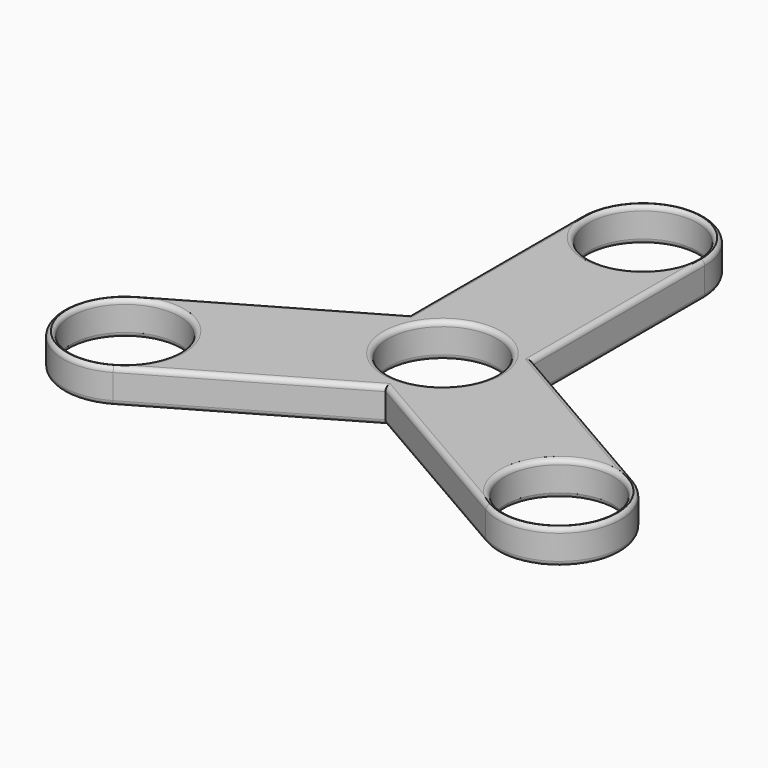
from build123d import *

# Parameters (mm, degrees)
F2_DEPTH      = 7
F1_R          = 11
F3_DEPTH      = 25.4
F4_T8_DEPTH   = 46.0831216351
F4_T13_DEPTH  = 46.0831216351
F4_T18_DEPTH  = 46.0831216351
F4_T23_DEPTH  = 46.0831216351
F4_T28_DEPTH  = 46.0831216351
F4_T37_DEPTH  = 46.0831216351
F4_T42_DEPTH  = 46.0831216351
F4_T51_DEPTH  = 46.0831216351
F4_T56_DEPTH  = 46.0831216351
F4_T59_ANGLE  = 180
F4_T61_ANGLE  = 180
F4_T63_ANGLE  = 180
F4_T67_DEPTH  = 46.0831216351
F4_T70_ANGLE  = 180
F4_T74_DEPTH  = 46.0831216351
F4_T77_ANGLE  = 180
F4_T81_DEPTH  = 46.0831216351
F4_T84_ANGLE  = 180
F4_T89_DEPTH  = 46.0831216351
F4_T93_DEPTH  = 46.0831216351
F4_T100_DEPTH = 46.0831216351
F4_T104_DEPTH = 46.0831216351
F4_T111_DEPTH = 46.0831216351
F4_T115_DEPTH = 46.0831216351
F4_T122_DEPTH = 46.0831216351
F4_T126_DEPTH = 46.0831216351
F4_T133_DEPTH = 46.0831216351
F4_T137_DEPTH = 46.0831216351
F4_T144_DEPTH = 46.0831216351
F4_T148_DEPTH = 46.0831216351
F5_R          = 1


# Not quite as in the source:
# - a fillet or chamfer that OpenCascade refuses, or shapes differently, is made with other operations: its cross-section is extruded or revolved along the edge and cut away or added


with BuildPart() as f2:
    # F0 (on Top) → F2 (new body)
    with BuildSketch(Plane.XY):
        with BuildLine():
            ThreePointArc((12.5, 50.8), (0, 63.3), (-12.5, 50.8))
            Line((-12.5, 50.8), (-12.5, 7.2168783649))
            Line((-12.5, 7.2168783649), (-50.2440905122, -14.5746824527))
            ThreePointArc((-50.2440905122, -14.5746824527), (-54.8194080596, -31.65), (-37.7440905122, -36.2253175473))
            Line((-37.7440905122, -36.2253175473), (0, -14.4337567297))
            Line((0, -14.4337567297), (37.7440905122, -36.2253175473))
            ThreePointArc((37.7440905122, -36.2253175473), (54.8194080596, -31.65), (50.2440905122, -14.5746824527))
            Line((50.2440905122, -14.5746824527), (12.5, 7.2168783649))
            Line((12.5, 7.2168783649), (12.5, 50.8))
        make_face()
    extrude(amount=F2_DEPTH)

    # F1 (on Top) → F3 (cut)
    with BuildSketch(Plane.XY):
        with Locations((0, 50.8)):
            Circle(F1_R)
        with Locations((-43.9940905122, -25.4)):
            Circle(F1_R)
        with Locations((43.9940905122, -25.4)):
            Circle(F1_R)
        Circle(F1_R)
    extrude(amount=F3_DEPTH, mode=Mode.SUBTRACT)

    # F4: fillet of radius 1 on 15 edges, made by hand

    # F4_s1 → F4_t2 (revolve, cut)
    with BuildSketch(Plane.XZ.offset(-50.8)):
        with BuildLine():
            ThreePointArc((12, 7), (11.2928932188, 6.7071067812), (11, 6))
            Line((11, 6), (11, 7))
            Line((11, 7), (12, 7))
        make_face()
    revolve(axis=Axis((0, 50.8, 7), (0, 0, -1)), mode=Mode.SUBTRACT)

    # F4_s3 → F4_t4 (revolve, cut)
    with BuildSketch(Plane.XZ.offset(-50.8)):
        with BuildLine():
            ThreePointArc((12, 0), (11.2928932188, 0.2928932188), (11, 1))
            Line((11, 1), (11, 0))
            Line((11, 0), (12, 0))
        make_face()
    revolve(axis=Axis((0, 50.8, 0), (0, 0, 1)), mode=Mode.SUBTRACT)


with BuildPart() as f4_tool6:
    # F4_s7 → F4_t8 (new body)
    with BuildSketch(Plane.XZ.offset(-50.8)):
        with BuildLine():
            ThreePointArc((-11.5, 0), (-12.2071067812, 0.2928932188), (-12.5, 1))
            Line((-12.5, 1), (-12.5, 0))
            Line((-12.5, 0), (-11.5, 0))
        make_face()
    extrude(amount=F4_T8_DEPTH)

    split(bisect_by=Plane(origin=(-6.25, 10.8253175473, 0), x_dir=(0, 0, 1), z_dir=(-0.5, 0.8660254038, 0)), keep=Keep.TOP)


with BuildPart() as f2_1:
    add(f2.part)

    # F4_t5: cut F4_tool6
    add(f4_tool6.part, mode=Mode.SUBTRACT)


with BuildPart() as f4_tool11:
    # F4_s12 → F4_t13 (new body)
    with BuildSketch(Plane.XZ.offset(-4.7168783649)):
        with BuildLine():
            ThreePointArc((11.5, 0), (12.2071067812, 0.2928932188), (12.5, 1))
            Line((12.5, 1), (12.5, 0))
            Line((12.5, 0), (11.5, 0))
        make_face()
    extrude(amount=-F4_T13_DEPTH)

    split(bisect_by=Plane(origin=(6.25, 10.8253175473, 0), x_dir=(0, 0, 1), z_dir=(0.5, 0.8660254038, 0)), keep=Keep.TOP)


with BuildPart() as f2_2:
    add(f2_1.part)

    # F4_t10: cut F4_tool11
    add(f4_tool11.part, mode=Mode.SUBTRACT)


with BuildPart() as f4_tool16:
    # F4_s17 → F4_t18 (new body)
    with BuildSketch(Plane.XZ.offset(-4.7168783649)):
        with BuildLine():
            ThreePointArc((11.5, 7), (12.2071067812, 6.7071067812), (12.5, 6))
            Line((12.5, 6), (12.5, 7))
            Line((12.5, 7), (11.5, 7))
        make_face()
    extrude(amount=-F4_T18_DEPTH)

    split(bisect_by=Plane(origin=(6.25, 10.8253175473, 0), x_dir=(0, 0, 1), z_dir=(0.5, 0.8660254038, 0)), keep=Keep.TOP)


with BuildPart() as f2_3:
    add(f2_2.part)

    # F4_t15: cut F4_tool16
    add(f4_tool16.part, mode=Mode.SUBTRACT)


with BuildPart() as f4_tool21:
    # F4_s22 → F4_t23 (new body)
    with BuildSketch(Plane(origin=(-4.0849364905, -2.3584391824, 0), x_dir=(0, 0, 1), z_dir=(-0.8660254038, -0.5, 0))):
        with BuildLine():
            ThreePointArc((0, 11.5), (0.2928932188, 12.2071067812), (1, 12.5))
            Line((1, 12.5), (0, 12.5))
            Line((0, 12.5), (0, 11.5))
        make_face()
    extrude(amount=F4_T23_DEPTH)

    split(bisect_by=Plane.YZ.offset(-12.5), keep=Keep.BOTTOM)


with BuildPart() as f2_4:
    add(f2_3.part)

    # F4_t20: cut F4_tool21
    add(f4_tool21.part, mode=Mode.SUBTRACT)


with BuildPart() as f4_tool26:
    # F4_s27 → F4_t28 (new body)
    with BuildSketch(Plane(origin=(-4.0849364905, -2.3584391824, 0), x_dir=(0, 0, 1), z_dir=(-0.8660254038, -0.5, 0))):
        with BuildLine():
            ThreePointArc((7, 11.5), (6.7071067812, 12.2071067812), (6, 12.5))
            Line((6, 12.5), (7, 12.5))
            Line((7, 12.5), (7, 11.5))
        make_face()
    extrude(amount=F4_T28_DEPTH)

    split(bisect_by=Plane.YZ.offset(-12.5), keep=Keep.BOTTOM)


with BuildPart() as f2_5:
    add(f2_4.part)

    # F4_t25: cut F4_tool26
    add(f4_tool26.part, mode=Mode.SUBTRACT)

    # F4_s30 → F4_t31 (revolve, cut)
    with BuildSketch(Plane.XZ.offset(25.4)):
        with BuildLine():
            ThreePointArc((-31.9940905122, 0), (-32.7011972934, 0.2928932188), (-32.9940905122, 1))
            Line((-32.9940905122, 1), (-32.9940905122, 0))
            Line((-32.9940905122, 0), (-31.9940905122, 0))
        make_face()
    revolve(axis=Axis((-43.9940905122, -25.4, 0), (0, 0, 1)), mode=Mode.SUBTRACT)

    # F4_s32 → F4_t33 (revolve, cut)
    with BuildSketch(Plane.XZ.offset(25.4)):
        with BuildLine():
            ThreePointArc((-31.9940905122, 7), (-32.7011972934, 6.7071067812), (-32.9940905122, 6))
            Line((-32.9940905122, 6), (-32.9940905122, 7))
            Line((-32.9940905122, 7), (-31.9940905122, 7))
        make_face()
    revolve(axis=Axis((-43.9940905122, -25.4, 7), (0, 0, -1)), mode=Mode.SUBTRACT)


with BuildPart() as f4_tool35:
    # F4_s36 → F4_t37 (new body)
    with BuildSketch(Plane(origin=(43.9940905122, -25.4, 0), x_dir=(0, 0, 1), z_dir=(-0.8660254038, 0.5, 0))):
        with BuildLine():
            ThreePointArc((7, 11.5), (6.7071067812, 12.2071067812), (6, 12.5))
            Line((6, 12.5), (7, 12.5))
            Line((7, 12.5), (7, 11.5))
        make_face()
    extrude(amount=F4_T37_DEPTH)

    split(bisect_by=Plane.YZ.offset(12.5), keep=Keep.TOP)


with BuildPart() as f2_6:
    add(f2_5.part)

    # F4_t34: cut F4_tool35
    add(f4_tool35.part, mode=Mode.SUBTRACT)


with BuildPart() as f4_tool40:
    # F4_s41 → F4_t42 (new body)
    with BuildSketch(Plane(origin=(4.0849364905, -2.3584391824, 0), x_dir=(0, 0, 1), z_dir=(0.8660254038, -0.5, 0))):
        with BuildLine():
            ThreePointArc((6, 12.5), (6.7071067812, 12.2071067812), (7, 11.5))
            Line((7, 11.5), (7, 12.5))
            Line((7, 12.5), (6, 12.5))
        make_face()
    extrude(amount=F4_T42_DEPTH)

    split(bisect_by=Plane(origin=(6.25, -10.8253175473, 0), x_dir=(0, 0, 1), z_dir=(0.5, -0.8660254038, 0)), keep=Keep.TOP)


with BuildPart() as f2_7:
    add(f2_6.part)

    # F4_t39: cut F4_tool40
    add(f4_tool40.part, mode=Mode.SUBTRACT)

    # F4_s44 → F4_t45 (revolve, cut)
    with BuildSketch(Plane.XZ.offset(25.4)):
        with BuildLine():
            ThreePointArc((55.9940905122, 7), (55.2869837311, 6.7071067812), (54.9940905122, 6))
            Line((54.9940905122, 6), (54.9940905122, 7))
            Line((54.9940905122, 7), (55.9940905122, 7))
        make_face()
    revolve(axis=Axis((43.9940905122, -25.4, 7), (0, 0, -1)), mode=Mode.SUBTRACT)

    # F4_s46 → F4_t47 (revolve, cut)
    with BuildSketch(Plane.XZ.offset(25.4)):
        with BuildLine():
            ThreePointArc((55.9940905122, 0), (55.2869837311, 0.2928932188), (54.9940905122, 1))
            Line((54.9940905122, 1), (54.9940905122, 0))
            Line((54.9940905122, 0), (55.9940905122, 0))
        make_face()
    revolve(axis=Axis((43.9940905122, -25.4, 0), (0, 0, 1)), mode=Mode.SUBTRACT)


with BuildPart() as f4_tool49:
    # F4_s50 → F4_t51 (new body)
    with BuildSketch(Plane(origin=(4.0849364905, -2.3584391824, 0), x_dir=(0, 0, 1), z_dir=(0.8660254038, -0.5, 0))):
        with BuildLine():
            ThreePointArc((1, 12.5), (0.2928932188, 12.2071067812), (0, 11.5))
            Line((0, 11.5), (0, 12.5))
            Line((0, 12.5), (1, 12.5))
        make_face()
    extrude(amount=F4_T51_DEPTH)

    split(bisect_by=Plane(origin=(6.25, -10.8253175473, 0), x_dir=(0, 0, 1), z_dir=(0.5, -0.8660254038, 0)), keep=Keep.TOP)


with BuildPart() as f2_8:
    add(f2_7.part)

    # F4_t48: cut F4_tool49
    add(f4_tool49.part, mode=Mode.SUBTRACT)


with BuildPart() as f4_tool54:
    # F4_s55 → F4_t56 (new body)
    with BuildSketch(Plane(origin=(43.9940905122, -25.4, 0), x_dir=(0, 0, 1), z_dir=(-0.8660254038, 0.5, 0))):
        with BuildLine():
            ThreePointArc((0, 11.5), (0.2928932188, 12.2071067812), (1, 12.5))
            Line((1, 12.5), (0, 12.5))
            Line((0, 12.5), (0, 11.5))
        make_face()
    extrude(amount=F4_T56_DEPTH)

    split(bisect_by=Plane.YZ.offset(12.5), keep=Keep.TOP)


with BuildPart() as f2_9:
    add(f2_8.part)

    # F4_t53: cut F4_tool54
    add(f4_tool54.part, mode=Mode.SUBTRACT)

    # F4_s58 → F4_t59 (revolve, cut)
    with BuildSketch(Plane(origin=(43.9940905122, -25.4, 0), x_dir=(0, 0, 1), z_dir=(-0.8660254038, 0.5, 0))):
        with BuildLine():
            ThreePointArc((0, -11.5), (0.2928932188, -12.2071067812), (1, -12.5))
            Line((1, -12.5), (0, -12.5))
            Line((0, -12.5), (0, -11.5))
        make_face()
    revolve(axis=Axis((43.9940905122, -25.4, 0), (0, 0, 1)), revolution_arc=F4_T59_ANGLE, mode=Mode.SUBTRACT)

    # F4_s60 → F4_t61 (revolve, cut)
    with BuildSketch(Plane(origin=(43.9940905122, -25.4, 0), x_dir=(0, 0, 1), z_dir=(-0.8660254038, 0.5, 0))):
        with BuildLine():
            ThreePointArc((7, -11.5), (6.7071067812, -12.2071067812), (6, -12.5))
            Line((6, -12.5), (7, -12.5))
            Line((7, -12.5), (7, -11.5))
        make_face()
    revolve(axis=Axis((43.9940905122, -25.4, 7), (0, 0, 1)), revolution_arc=F4_T61_ANGLE, mode=Mode.SUBTRACT)

    # F4_s62 → F4_t63 (revolve, cut)
    with BuildSketch(Plane(origin=(-43.9940905122, -25.4, 0), x_dir=(0, 0, 1), z_dir=(0.8660254038, 0.5, 0))):
        with BuildLine():
            ThreePointArc((6, -12.5), (6.7071067812, -12.2071067812), (7, -11.5))
            Line((7, -11.5), (7, -12.5))
            Line((7, -12.5), (6, -12.5))
        make_face()
    revolve(axis=Axis((-43.9940905122, -25.4, 7), (0, 0, 1)), revolution_arc=F4_T63_ANGLE, mode=Mode.SUBTRACT)


with BuildPart() as f4_tool65:
    # F4_s66 → F4_t67 (new body)
    with BuildSketch(Plane(origin=(-43.9940905122, -25.4, 0), x_dir=(0, 0, 1), z_dir=(0.8660254038, 0.5, 0))):
        with BuildLine():
            ThreePointArc((6, 12.5), (6.7071067812, 12.2071067812), (7, 11.5))
            Line((7, 11.5), (7, 12.5))
            Line((7, 12.5), (6, 12.5))
        make_face()
    extrude(amount=F4_T67_DEPTH)

    split(bisect_by=Plane(origin=(-6.25, -10.8253175473, 0), x_dir=(0, 0, 1), z_dir=(-0.5, -0.8660254038, 0)), keep=Keep.TOP)


with BuildPart() as f2_10:
    add(f2_9.part)

    # F4_t64: cut F4_tool65
    add(f4_tool65.part, mode=Mode.SUBTRACT)

    # F4_s69 → F4_t70 (revolve, cut)
    with BuildSketch(Plane(origin=(-43.9940905122, -25.4, 0), x_dir=(0, 0, 1), z_dir=(0.8660254038, 0.5, 0))):
        with BuildLine():
            ThreePointArc((1, -12.5), (0.2928932188, -12.2071067812), (0, -11.5))
            Line((0, -11.5), (0, -12.5))
            Line((0, -12.5), (1, -12.5))
        make_face()
    revolve(axis=Axis((-43.9940905122, -25.4, 0), (0, 0, 1)), revolution_arc=F4_T70_ANGLE, mode=Mode.SUBTRACT)


with BuildPart() as f4_tool72:
    # F4_s73 → F4_t74 (new body)
    with BuildSketch(Plane(origin=(-43.9940905122, -25.4, 0), x_dir=(0, 0, 1), z_dir=(0.8660254038, 0.5, 0))):
        with BuildLine():
            ThreePointArc((1, 12.5), (0.2928932188, 12.2071067812), (0, 11.5))
            Line((0, 11.5), (0, 12.5))
            Line((0, 12.5), (1, 12.5))
        make_face()
    extrude(amount=F4_T74_DEPTH)

    split(bisect_by=Plane(origin=(-6.25, -10.8253175473, 0), x_dir=(0, 0, 1), z_dir=(-0.5, -0.8660254038, 0)), keep=Keep.TOP)


with BuildPart() as f2_11:
    add(f2_10.part)

    # F4_t71: cut F4_tool72
    add(f4_tool72.part, mode=Mode.SUBTRACT)

    # F4_s76 → F4_t77 (revolve, cut)
    with BuildSketch(Plane.XZ.offset(-50.8)):
        with BuildLine():
            ThreePointArc((11.5, 7), (12.2071067812, 6.7071067812), (12.5, 6))
            Line((12.5, 6), (12.5, 7))
            Line((12.5, 7), (11.5, 7))
        make_face()
    revolve(axis=Axis((0, 50.8, 7), (0, 0, 1)), revolution_arc=F4_T77_ANGLE, mode=Mode.SUBTRACT)


with BuildPart() as f4_tool79:
    # F4_s80 → F4_t81 (new body)
    with BuildSketch(Plane.XZ.offset(-50.8)):
        with BuildLine():
            ThreePointArc((-11.5, 7), (-12.2071067812, 6.7071067812), (-12.5, 6))
            Line((-12.5, 6), (-12.5, 7))
            Line((-12.5, 7), (-11.5, 7))
        make_face()
    extrude(amount=F4_T81_DEPTH)

    split(bisect_by=Plane(origin=(-6.25, 10.8253175473, 0), x_dir=(0, 0, 1), z_dir=(-0.5, 0.8660254038, 0)), keep=Keep.TOP)


with BuildPart() as f2_12:
    add(f2_11.part)

    # F4_t78: cut F4_tool79
    add(f4_tool79.part, mode=Mode.SUBTRACT)

    # F4_s83 → F4_t84 (revolve, cut)
    with BuildSketch(Plane.XZ.offset(-50.8)):
        with BuildLine():
            ThreePointArc((11.5, 0), (12.2071067812, 0.2928932188), (12.5, 1))
            Line((12.5, 1), (12.5, 0))
            Line((12.5, 0), (11.5, 0))
        make_face()
    revolve(axis=Axis((0, 50.8, 0), (0, 0, 1)), revolution_arc=F4_T84_ANGLE, mode=Mode.SUBTRACT)


with BuildPart() as f4_tool87:
    # F4_s88 → F4_t89 (new body)
    with BuildSketch(Plane(origin=(-4.0849364905, -2.3584391824, 0), x_dir=(0, 0, 1), z_dir=(-0.8660254038, -0.5, 0))):
        with BuildLine():
            ThreePointArc((0, 11.5), (0.2928932188, 12.2071067812), (1, 12.5))
            Line((1, 12.5), (0, 12.5))
            Line((0, 12.5), (0, 11.5))
        make_face()
    extrude(amount=F4_T89_DEPTH)

    split(bisect_by=Plane.YZ.offset(-12.5), keep=Keep.TOP)


with BuildPart() as f4_tool91:
    # F4_s92 → F4_t93 (new body)
    with BuildSketch(Plane.XZ.offset(-50.8)):
        with BuildLine():
            ThreePointArc((-11.5, 0), (-12.2071067812, 0.2928932188), (-12.5, 1))
            Line((-12.5, 1), (-12.5, 0))
            Line((-12.5, 0), (-11.5, 0))
        make_face()
    extrude(amount=F4_T93_DEPTH)

    split(bisect_by=Plane(origin=(-6.25, 10.8253175473, 0), x_dir=(0, 0, 1), z_dir=(0.5, -0.8660254038, 0)), keep=Keep.TOP)


with BuildPart() as f4_tool87_1:
    add(f4_tool87.part)

    # F4_t95: intersect F4_tool91
    add(f4_tool91.part, mode=Mode.INTERSECT)


with BuildPart() as f2_13:
    add(f2_12.part)

    # F4_t85: cut F4_tool87
    add(f4_tool87_1.part, mode=Mode.SUBTRACT)


with BuildPart() as f4_tool98:
    # F4_s99 → F4_t100 (new body)
    with BuildSketch(Plane(origin=(43.9940905122, -25.4, 0), x_dir=(0, 0, 1), z_dir=(-0.8660254038, 0.5, 0))):
        with BuildLine():
            ThreePointArc((0, 11.5), (0.2928932188, 12.2071067812), (1, 12.5))
            Line((1, 12.5), (0, 12.5))
            Line((0, 12.5), (0, 11.5))
        make_face()
    extrude(amount=F4_T100_DEPTH)

    split(bisect_by=Plane.YZ.offset(12.5), keep=Keep.BOTTOM)


with BuildPart() as f4_tool102:
    # F4_s103 → F4_t104 (new body)
    with BuildSketch(Plane.XZ.offset(-4.7168783649)):
        with BuildLine():
            ThreePointArc((11.5, 0), (12.2071067812, 0.2928932188), (12.5, 1))
            Line((12.5, 1), (12.5, 0))
            Line((12.5, 0), (11.5, 0))
        make_face()
    extrude(amount=-F4_T104_DEPTH)

    split(bisect_by=Plane(origin=(6.25, 10.8253175473, 0), x_dir=(0, 0, 1), z_dir=(-0.5, -0.8660254038, 0)), keep=Keep.TOP)


with BuildPart() as f4_tool98_1:
    add(f4_tool98.part)

    # F4_t106: intersect F4_tool102
    add(f4_tool102.part, mode=Mode.INTERSECT)


with BuildPart() as f2_14:
    add(f2_13.part)

    # F4_t96: cut F4_tool98
    add(f4_tool98_1.part, mode=Mode.SUBTRACT)


with BuildPart() as f4_tool109:
    # F4_s110 → F4_t111 (new body)
    with BuildSketch(Plane(origin=(43.9940905122, -25.4, 0), x_dir=(0, 0, 1), z_dir=(-0.8660254038, 0.5, 0))):
        with BuildLine():
            ThreePointArc((7, 11.5), (6.7071067812, 12.2071067812), (6, 12.5))
            Line((6, 12.5), (7, 12.5))
            Line((7, 12.5), (7, 11.5))
        make_face()
    extrude(amount=F4_T111_DEPTH)

    split(bisect_by=Plane.YZ.offset(12.5), keep=Keep.BOTTOM)


with BuildPart() as f4_tool113:
    # F4_s114 → F4_t115 (new body)
    with BuildSketch(Plane.XZ.offset(-4.7168783649)):
        with BuildLine():
            ThreePointArc((11.5, 7), (12.2071067812, 6.7071067812), (12.5, 6))
            Line((12.5, 6), (12.5, 7))
            Line((12.5, 7), (11.5, 7))
        make_face()
    extrude(amount=-F4_T115_DEPTH)

    split(bisect_by=Plane(origin=(6.25, 10.8253175473, 0), x_dir=(0, 0, 1), z_dir=(-0.5, -0.8660254038, 0)), keep=Keep.TOP)


with BuildPart() as f4_tool109_1:
    add(f4_tool109.part)

    # F4_t117: intersect F4_tool113
    add(f4_tool113.part, mode=Mode.INTERSECT)


with BuildPart() as f2_15:
    add(f2_14.part)

    # F4_t107: cut F4_tool109
    add(f4_tool109_1.part, mode=Mode.SUBTRACT)


with BuildPart() as f4_tool120:
    # F4_s121 → F4_t122 (new body)
    with BuildSketch(Plane(origin=(-4.0849364905, -2.3584391824, 0), x_dir=(0, 0, 1), z_dir=(-0.8660254038, -0.5, 0))):
        with BuildLine():
            ThreePointArc((7, 11.5), (6.7071067812, 12.2071067812), (6, 12.5))
            Line((6, 12.5), (7, 12.5))
            Line((7, 12.5), (7, 11.5))
        make_face()
    extrude(amount=F4_T122_DEPTH)

    split(bisect_by=Plane.YZ.offset(-12.5), keep=Keep.TOP)


with BuildPart() as f4_tool124:
    # F4_s125 → F4_t126 (new body)
    with BuildSketch(Plane.XZ.offset(-50.8)):
        with BuildLine():
            ThreePointArc((-11.5, 7), (-12.2071067812, 6.7071067812), (-12.5, 6))
            Line((-12.5, 6), (-12.5, 7))
            Line((-12.5, 7), (-11.5, 7))
        make_face()
    extrude(amount=F4_T126_DEPTH)

    split(bisect_by=Plane(origin=(-6.25, 10.8253175473, 0), x_dir=(0, 0, 1), z_dir=(0.5, -0.8660254038, 0)), keep=Keep.TOP)


with BuildPart() as f4_tool120_1:
    add(f4_tool120.part)

    # F4_t128: intersect F4_tool124
    add(f4_tool124.part, mode=Mode.INTERSECT)


with BuildPart() as f2_16:
    add(f2_15.part)

    # F4_t118: cut F4_tool120
    add(f4_tool120_1.part, mode=Mode.SUBTRACT)


with BuildPart() as f4_tool131:
    # F4_s132 → F4_t133 (new body)
    with BuildSketch(Plane(origin=(-43.9940905122, -25.4, 0), x_dir=(0, 0, 1), z_dir=(0.8660254038, 0.5, 0))):
        with BuildLine():
            ThreePointArc((6, 12.5), (6.7071067812, 12.2071067812), (7, 11.5))
            Line((7, 11.5), (7, 12.5))
            Line((7, 12.5), (6, 12.5))
        make_face()
    extrude(amount=F4_T133_DEPTH)

    split(bisect_by=Plane(origin=(-6.25, -10.8253175473, 0), x_dir=(0, 0, 1), z_dir=(0.5, 0.8660254038, 0)), keep=Keep.TOP)


with BuildPart() as f4_tool135:
    # F4_s136 → F4_t137 (new body)
    with BuildSketch(Plane(origin=(4.0849364905, -2.3584391824, 0), x_dir=(0, 0, 1), z_dir=(0.8660254038, -0.5, 0))):
        with BuildLine():
            ThreePointArc((6, 12.5), (6.7071067812, 12.2071067812), (7, 11.5))
            Line((7, 11.5), (7, 12.5))
            Line((7, 12.5), (6, 12.5))
        make_face()
    extrude(amount=F4_T137_DEPTH)

    split(bisect_by=Plane(origin=(6.25, -10.8253175473, 0), x_dir=(0, 0, 1), z_dir=(-0.5, 0.8660254038, 0)), keep=Keep.TOP)


with BuildPart() as f4_tool131_1:
    add(f4_tool131.part)

    # F4_t139: intersect F4_tool135
    add(f4_tool135.part, mode=Mode.INTERSECT)


with BuildPart() as f2_17:
    add(f2_16.part)

    # F4_t129: cut F4_tool131
    add(f4_tool131_1.part, mode=Mode.SUBTRACT)


with BuildPart() as f4_tool142:
    # F4_s143 → F4_t144 (new body)
    with BuildSketch(Plane(origin=(-43.9940905122, -25.4, 0), x_dir=(0, 0, 1), z_dir=(0.8660254038, 0.5, 0))):
        with BuildLine():
            ThreePointArc((1, 12.5), (0.2928932188, 12.2071067812), (0, 11.5))
            Line((0, 11.5), (0, 12.5))
            Line((0, 12.5), (1, 12.5))
        make_face()
    extrude(amount=F4_T144_DEPTH)

    split(bisect_by=Plane(origin=(-6.25, -10.8253175473, 0), x_dir=(0, 0, 1), z_dir=(0.5, 0.8660254038, 0)), keep=Keep.TOP)


with BuildPart() as f4_tool146:
    # F4_s147 → F4_t148 (new body)
    with BuildSketch(Plane(origin=(4.0849364905, -2.3584391824, 0), x_dir=(0, 0, 1), z_dir=(0.8660254038, -0.5, 0))):
        with BuildLine():
            ThreePointArc((1, 12.5), (0.2928932188, 12.2071067812), (0, 11.5))
            Line((0, 11.5), (0, 12.5))
            Line((0, 12.5), (1, 12.5))
        make_face()
    extrude(amount=F4_T148_DEPTH)

    split(bisect_by=Plane(origin=(6.25, -10.8253175473, 0), x_dir=(0, 0, 1), z_dir=(-0.5, 0.8660254038, 0)), keep=Keep.TOP)


with BuildPart() as f4_tool142_1:
    add(f4_tool142.part)

    # F4_t150: intersect F4_tool146
    add(f4_tool146.part, mode=Mode.INTERSECT)


with BuildPart() as f2_18:
    add(f2_17.part)

    # F4_t140: cut F4_tool142
    add(f4_tool142_1.part, mode=Mode.SUBTRACT)

    # F5
    f5_edges = [f2_18.edges().sort_by_distance(p)[0] for p in [
        (-11, 0, 7),
        (-11, 0, 0),
    ]]
    fillet(f5_edges, radius=F5_R)


solid = f2_18.part
